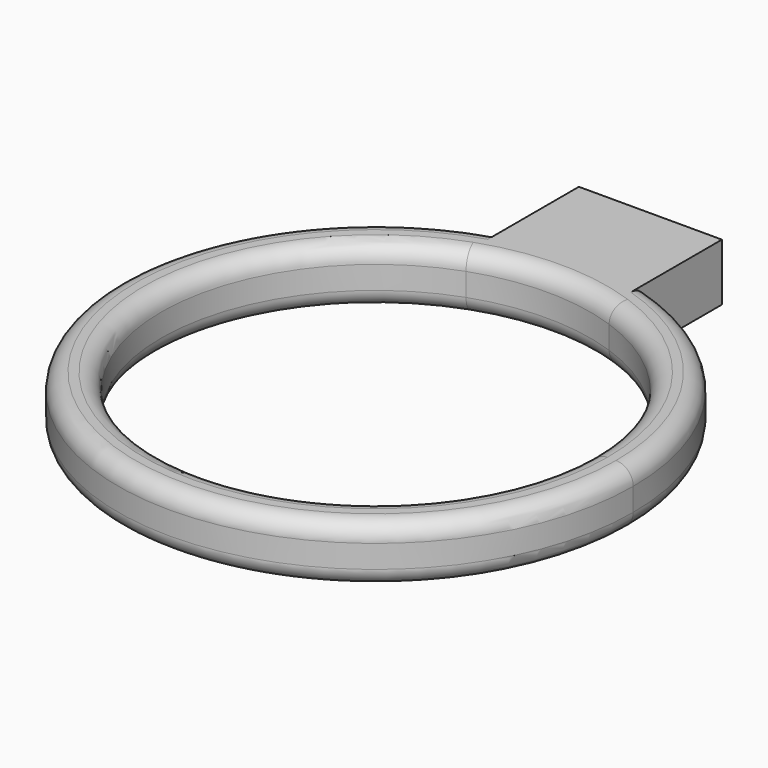
from build123d import *

# Parameters (mm, degrees)
F1_DEPTH = 2
F2_R     = 0.6


# Not quite as in the source:
# - a feature names something its author has since deleted; it is built from what else it names


with BuildPart() as f1:
    # F0 (on Top) → F1 (new body)
    with BuildSketch(Plane.XY):
        with BuildLine():
            ThreePointArc((2.5, 7.0710678119), (6.123724357, 4.3301270189), (7.5, 0))
            ThreePointArc((7.5, 0), (-4.3301270189, -6.123724357), (-2.5, 7.0710678119))
            Line((-2.5, 7.0710678119), (-2.5, 8.6458082329))
            ThreePointArc((-2.5, 8.6458082329), (-5.4083269132, -7.193747285), (9, 0))
            ThreePointArc((9, 0), (7.193747285, 5.4083269132), (2.5, 8.6458082329))
            Line((2.5, 8.6458082329), (2.5, 7.0710678119))
        make_face()
        with BuildLine():
            ThreePointArc((-2.5, 7.0710678119), (0, 7.5), (2.5, 7.0710678119))
            Line((2.5, 7.0710678119), (2.5, 8.6458082329))
            ThreePointArc((2.5, 8.6458082329), (0, 9), (-2.5, 8.6458082329))
            Line((-2.5, 8.6458082329), (-2.5, 7.0710678119))
        make_face()
        with BuildLine():
            ThreePointArc((-2.5, 8.6458082329), (0, 9), (2.5, 8.6458082329))
            Line((2.5, 8.6458082329), (2.5, 12))
            Line((2.5, 12), (-2.5, 12))
            Line((-2.5, 12), (-2.5, 8.6458082329))
        make_face()
    extrude(amount=F1_DEPTH)

    # F2
    f2_edges = [f1.edges().sort_by_distance(p)[0] for p in [
        (0, -9, 0),
        (0, -9, 2),
        (-7.5, 0, 2),
        (-7.5, 0, 0),
    ]]
    fillet(f2_edges, radius=F2_R)


solid = f1.part
